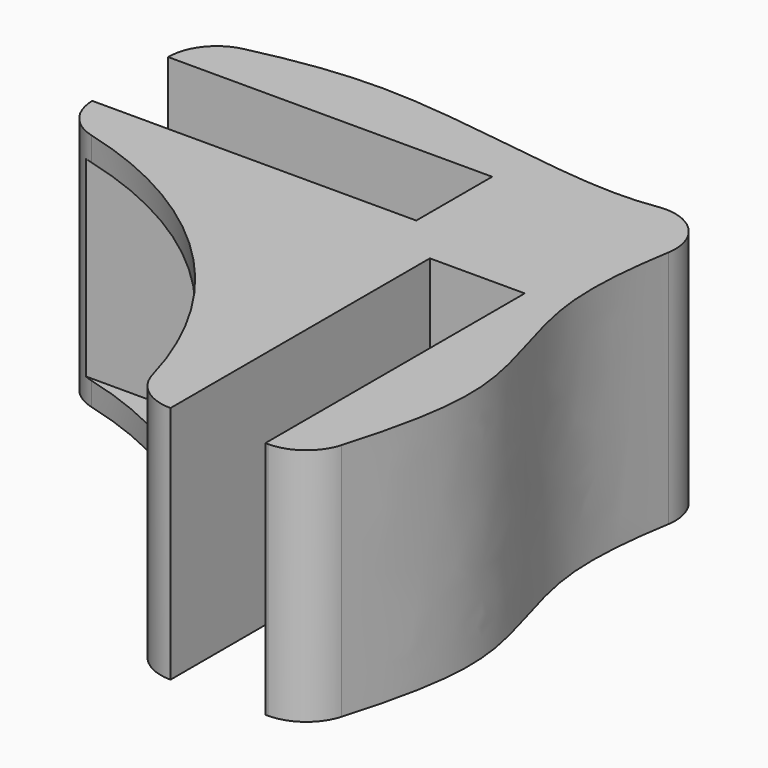
from build123d import *

# Parameters (mm, degrees)
F1_DEPTH    = 25
F2_W        = 30.2227726206
F2_H        = 20.068306243
F3_DEPTH    = 34
F4_T1_DEPTH = 45.2364697276
F5_R        = 5


# Not quite as in the source:
# - a fillet or chamfer that OpenCascade refuses, or shapes differently, is made with other operations: its cross-section is extruded or revolved along the edge and cut away or added


with BuildPart() as f1:
    # F0 (on Top) → F1 (new body)
    with BuildSketch(Plane.XY):
        with BuildLine():
            Line((-4.959, -9.4801727682), (4.959, -9.4801727682))
            Line((4.959, -9.4801727682), (4.959, -43.3722550981))
            Line((4.959, -43.3722550981), (8.959, -43.3722550981))
            add(Edge.make_bspline(
                [(8.959, -43.3722550981), (10.9444993843, -36.8281108572), (14.7331593025, -24.340805557), (6.9032731799, -9.0055840914), (9.6423102918, 4.2067701187), (11.0949236172, 11.2137733098)],
                knots=[0, 0, 0, 0, 0.3408719694, 0.6504398731, 1, 1, 1, 1], degree=3))
            add(Edge.make_bspline(
                [(-43.8664413989, 8.959), (-38.2964370805, 10.3608151634), (-26.1129886059, 13.4270502754), (-0.196589781, 7.3008338793), (7.8789436209, 10.0993137603), (11.0949236172, 11.2137733098)],
                knots=[0, 0, 0, 0, 0.3363503338, 0.7357098355, 1, 1, 1, 1], degree=3))
            Line((-43.8664413989, 8.959), (-43.8664413989, 4.959))
            Line((-43.8664413989, 4.959), (-10, 4.959))
            Line((-10, 4.959), (-10, -4.959))
            Line((-10, -4.959), (-43.8664413989, -4.959))
            Line((-43.8664413989, -4.959), (-43.8664413989, -8.959))
            ThreePointArc((-43.8664413989, -8.959), (-22.3244394728, -19.3298404084), (-9.7910396518, -39.6897536373))
            ThreePointArc((-9.7910396518, -39.6897536373), (-8.0019231601, -42.3463897646), (-4.9677422736, -43.3722550981))
            Line((-4.9677422736, -43.3722550981), (-4.959, -43.3722550981))
            Line((-4.959, -43.3722550981), (-4.959, -9.4801727682))
        make_face()
    extrude(amount=F1_DEPTH)

    # F2 (on face) → F3 (cut)
    with BuildSketch(Plane(origin=(-43.8664413989, 0, 0), x_dir=(0, -1, 0), z_dir=(-1, 0, 0))):
        with Locations((24.5702010579, 12.4597531976)):
            Rectangle(F2_W, F2_H)
    extrude(amount=-F3_DEPTH, mode=Mode.SUBTRACT)

    # F4: fillet of radius 5 on 1 edges, made by hand

    # F4_s2 → F4_t1 (cut)
    with BuildSketch(Plane.XY.offset(-10.1182348638)):
        with BuildLine():
            ThreePointArc((-40.1210831358, -9.7517343717), (-42.8207560477, -7.971672665), (-43.8664413989, -4.9117060545))
            Line((-43.8664413989, -4.9117060545), (-43.8664413989, -8.959))
            ThreePointArc((-43.8664413989, -8.959), (-41.9848306621, -9.3131688624), (-40.1210831358, -9.7517343717))
        make_face()
    extrude(amount=F4_T1_DEPTH, mode=Mode.SUBTRACT)

    # F5
    f5_edges = [f1.edges().sort_by_distance(p)[0] for p in [
        (8.959, -43.372255, 12.5),
        (11.094924, 11.213773, 12.5),
        (-43.866441, 8.959, 12.5),
    ]]
    fillet(f5_edges, radius=F5_R)


solid = f1.part
